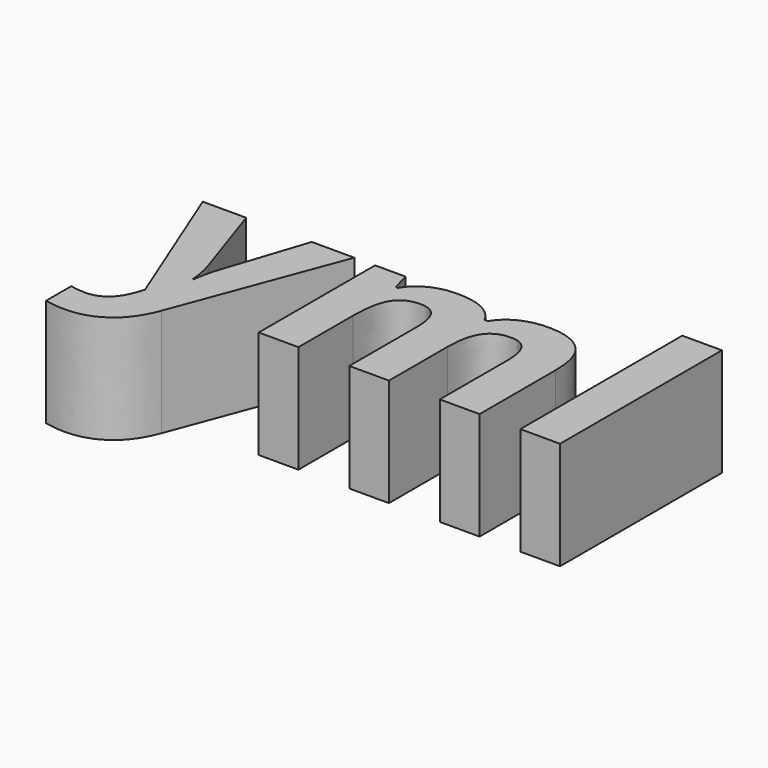
from build123d import *

# Parameters (mm, degrees)
F0_TEXT_SIZE = 61.7299642828
F1_DEPTH     = 25


# Not quite as in the source:
# - Text() gives the source's letters only with a copy of the font that has no kerning and outlines rounded to 1/6400 em; it was checked with that copy


with BuildPart() as f1:
    # F0 (on Top) → F1 (new body)
    with BuildSketch(Plane.XY):
        with Locations((0, -44.4455742836)):
            Text('yml', F0_TEXT_SIZE, font='Open Sans', font_style=FontStyle.BOLD, text_align=(TextAlign.LEFT, TextAlign.BOTTOM))
    extrude(amount=F1_DEPTH)


solid = f1.part
